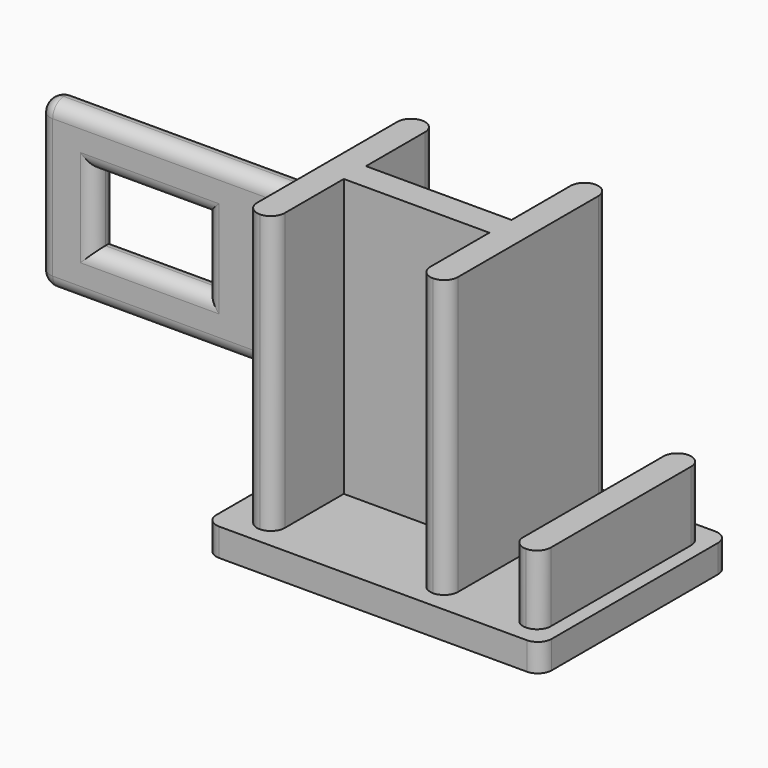
from build123d import *

# Parameters (mm, degrees)
F0_W     = 24.2
F0_H     = 17
F0_W_2   = 2
F0_H_2   = 14.65
F0_W_3   = 10.5
F0_H_3   = 1
F1_DEPTH = 2
F2_DEPTH = 20
F3_DEPTH = 5
F4_W     = 2
F4_H     = 12
F5_DEPTH = 20
F6_W     = 8
F6_H     = 5
F7_DEPTH = 25
F8_R     = 0.99999


# Not quite as in the source:
# - a fillet or chamfer is up to 0.001 mm smaller than in the source, because OpenCascade refuses the exact size


with BuildPart() as f1:
    # F0 (on Top) → F1 (new body)
    with BuildSketch(Plane.XY):
        Rectangle(F0_W, F0_H)
        Polygon((-10.1, 7.325), (-8.1, 7.325), (-8.1, 1), (2.4, 1), (2.4, 7.325), (4.4, 7.325), (4.4, -7.325), (2.4, -7.325), (2.4, -1), (-8.1, -1), (-8.1, -7.325), (-10.1, -7.325), align=None, mode=Mode.SUBTRACT)
        with Locations((10.1, 0)):
            Rectangle(F0_W_2, F0_H_2, mode=Mode.SUBTRACT)
        Polygon((-8.1, 1), (-8.1, 7.325), (-10.1, 7.325), (-10.1, -7.325), (-8.1, -7.325), (-8.1, -1), (-8.1, 0), align=None)
        Polygon((2.4, 7.325), (2.4, 1), (2.4, 0), (2.4, -1), (2.4, -7.325), (4.4, -7.325), (4.4, 7.325), align=None)
        with Locations((10.1, 0)):
            Rectangle(F0_W_2, F0_H_2)
        with Locations((-2.85, -0.5)):
            Rectangle(F0_W_3, F0_H_3)
        with Locations((-2.85, 0.5)):
            Rectangle(F0_W_3, F0_H_3)
    extrude(amount=-F1_DEPTH)

    # F0 (on Top) → F2 (join)
    with BuildSketch(Plane.XY):
        Polygon((-8.1, 1), (-8.1, 7.325), (-10.1, 7.325), (-10.1, -7.325), (-8.1, -7.325), (-8.1, -1), (-8.1, 0), align=None)
        with Locations((-2.85, 0.5)):
            Rectangle(F0_W_3, F0_H_3)
        Polygon((2.4, 7.325), (2.4, 1), (2.4, 0), (2.4, -1), (2.4, -7.325), (4.4, -7.325), (4.4, 7.325), align=None)
        with Locations((-2.85, -0.5)):
            Rectangle(F0_W_3, F0_H_3)
    extrude(amount=F2_DEPTH)

    # F0 (on Top) → F3 (join)
    with BuildSketch(Plane.XY):
        with Locations((10.1, 0)):
            Rectangle(F0_W_2, F0_H_2)
    extrude(amount=F3_DEPTH)

    # F4 (on face) → F5 (join)
    with BuildSketch(Plane(origin=(-10.1, 0, 0), x_dir=(0, -1, 0), z_dir=(-1, 0, 0))):
        with Locations((0, 12)):
            Rectangle(F4_W, F4_H)
    extrude(amount=F5_DEPTH)

    # F6 (on face) → F7 (cut)
    with BuildSketch(Plane(origin=(0, 1, 0), x_dir=(-1, 0, 0), z_dir=(0, 1, 0))):
        with Locations((22.1, 12)):
            Rectangle(F6_W, F6_H)
    extrude(amount=-F7_DEPTH, mode=Mode.SUBTRACT)

    # F8 (radius 1 in the source; OpenCascade refuses exactly that, so slightly less here)
    f8_edges = [f1.edges().sort_by_distance(p)[0] for p in [
        (-12.1, -8.5, -1),
        (-12.1, 8.5, -1),
        (12.1, -8.5, -1),
        (12.1, 8.5, -1),
        (11.1, -7.325, 2.5),
        (9.1, -7.325, 2.5),
        (11.1, 7.325, 2.5),
        (9.1, 7.325, 2.5),
        (2.4, -7.325, 10),
        (4.4, -7.325, 10),
        (-8.1, -7.325, 10),
        (-10.1, -7.325, 10),
        (-10.1, 7.325, 10),
        (-8.1, 7.325, 10),
        (2.4, 7.325, 10),
        (4.4, 7.325, 10),
        (-20.1, 1, 18),
        (-30.1, 1, 12),
        (-30.1, -1, 12),
        (-20.1, 1, 6),
        (-30.1, 0, 6),
        (-30.1, 0, 18),
        (-20.1, -1, 18),
        (-20.1, -1, 6),
        (-22.1, 1, 14.5),
        (-18.1, 1, 12),
        (-22.1, 1, 9.5),
        (-26.1, 1, 12),
        (-18.1, -1, 12),
        (-22.1, -1, 9.5),
        (-22.1, -1, 14.5),
        (-26.1, -1, 12),
    ]]
    fillet(f8_edges, radius=F8_R)


solid = f1.part
